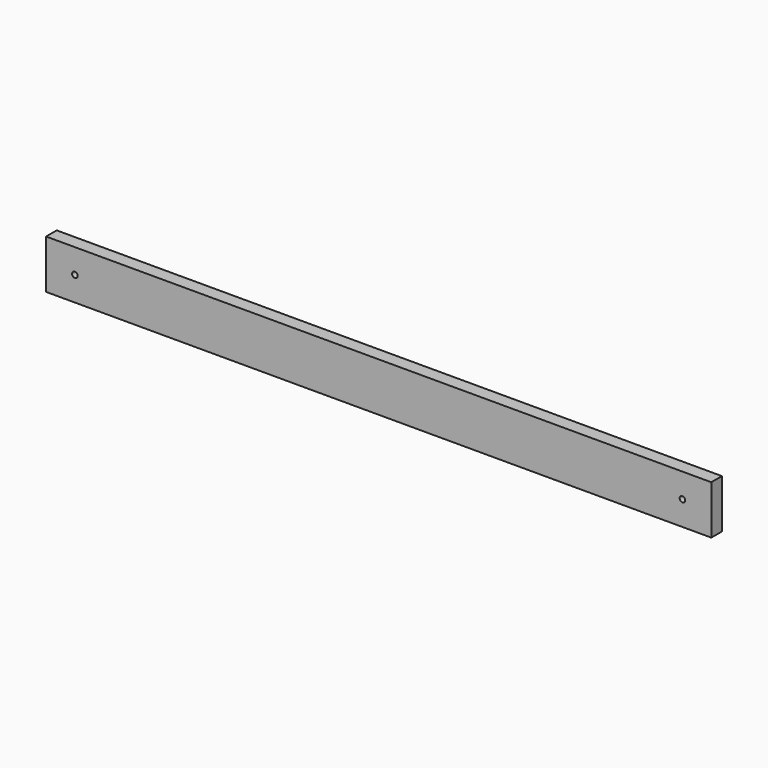
from build123d import *

# Parameters (mm, degrees)
F0_W     = 139.7
F0_H     = 38.1
F1_DEPTH = 1905
F2_ANGLE = 90
F4_D     = 15.875


with BuildPart() as f1:
    # F0 (on Top) → F1 (new body)
    with BuildSketch(Plane.XY):
        with Locations((69.85, 19.05)):
            Rectangle(F0_W, F0_H)
    extrude(amount=F1_DEPTH)


with BuildPart() as f1_1:
    # F2: moved
    add(f1.part.rotate(Axis((0, 19.05, 0), (0, -1, 0)), F2_ANGLE))

    # F4 (through all)
    with Locations(Plane.XZ):
        with Locations((-82.55, 69.85), (-1822.45, 69.85)):
            Hole(F4_D / 2)


solid = f1_1.part
